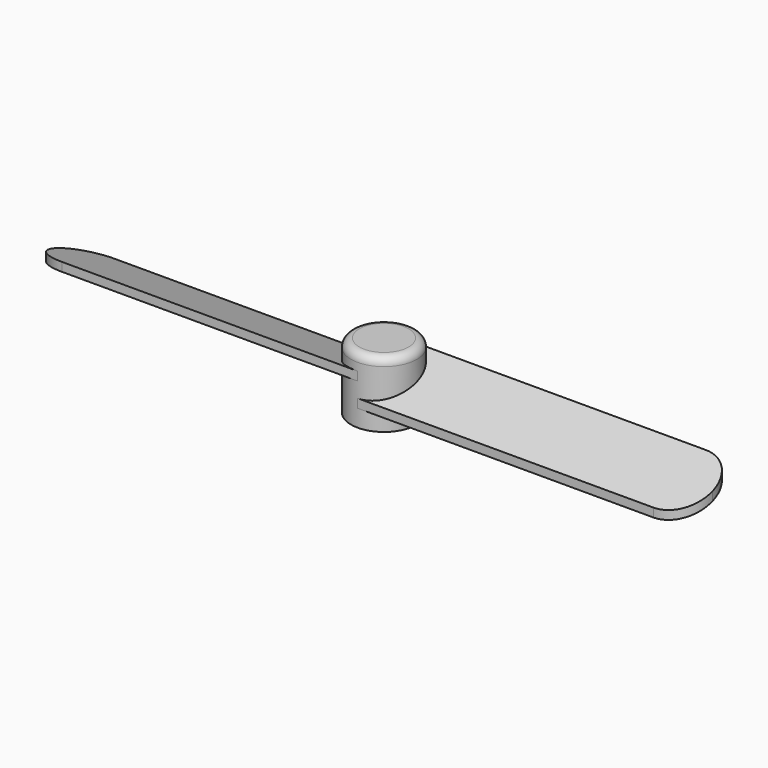
from build123d import *

# Parameters (mm, degrees)
F0_R        = 2
F1_DEPTH    = 4
F3_DEPTH    = 20
F5_DEPTH    = 20
F6_T1_DEPTH = 10.5320888862
F6_T3_DEPTH = 10.5320888862
F7_R        = 0.5
F8_R        = 0.25
F9_DEPTH    = 3


# Not quite as in the source:
# - a fillet or chamfer that OpenCascade refuses, or shapes differently, is made with other operations: its cross-section is extruded or revolved along the edge and cut away or added


with BuildPart() as f1:
    # F0 (on Top) → F1 (new body)
    with BuildSketch(Plane.XY):
        Circle(F0_R)
    extrude(amount=F1_DEPTH)

    # F2 (on Right) → F3 (join)
    with BuildSketch(Plane.YZ):
        Polygon((2, 3.0320888862), (-2, 1.5762079492), (-2, 1.0441190629), (2, 2.5), align=None)
    extrude(amount=F3_DEPTH)

    # F4 (on Right) → F5 (join)
    with BuildSketch(Plane.YZ):
        Polygon((2, 1.0441190629), (2, 1.5762079492), (-2, 3.0320888862), (-2, 2.5), align=None)
    extrude(amount=-F5_DEPTH)

    # F6: fillet of radius 2 on 4 edges, made by hand

    # F6_s2 → F6_t1 (cut)
    with BuildSketch(Plane.XY.offset(-3.9558809371)):
        with BuildLine():
            ThreePointArc((-18, 2), (-19.4142135624, 1.4142135624), (-20, 0))
            Line((-20, 0), (-20, 2))
            Line((-20, 2), (-18, 2))
        make_face()
        with BuildLine():
            ThreePointArc((18, -2), (19.4142135624, -1.4142135624), (20, 0))
            Line((20, 0), (20, -2))
            Line((20, -2), (18, -2))
        make_face()
    extrude(amount=F6_T1_DEPTH, mode=Mode.SUBTRACT)

    # F6_s4 → F6_t3 (cut)
    with BuildSketch(Plane.XY.offset(-2.5)):
        with BuildLine():
            ThreePointArc((-18, -2), (-19.4142135624, -1.4142135624), (-20, 0))
            Line((-20, 0), (-20, -2))
            Line((-20, -2), (-18, -2))
        make_face()
        with BuildLine():
            ThreePointArc((18, 2), (19.4142135624, 1.4142135624), (20, 0))
            Line((20, 0), (20, 2))
            Line((20, 2), (18, 2))
        make_face()
    extrude(amount=F6_T3_DEPTH, mode=Mode.SUBTRACT)

    # F7
    f7_edges = [f1.edges().sort_by_distance(p)[0] for p in [
        (-2, 0, 4),
    ]]
    fillet(f7_edges, radius=F7_R)

    # F8 (on face) → F9 (cut)
    with BuildSketch(Plane(origin=(0, 0, 0), x_dir=(1, 0, 0), z_dir=(0, 0, -1))):
        Circle(F8_R)
    extrude(amount=-F9_DEPTH, mode=Mode.SUBTRACT)


solid = f1.part
